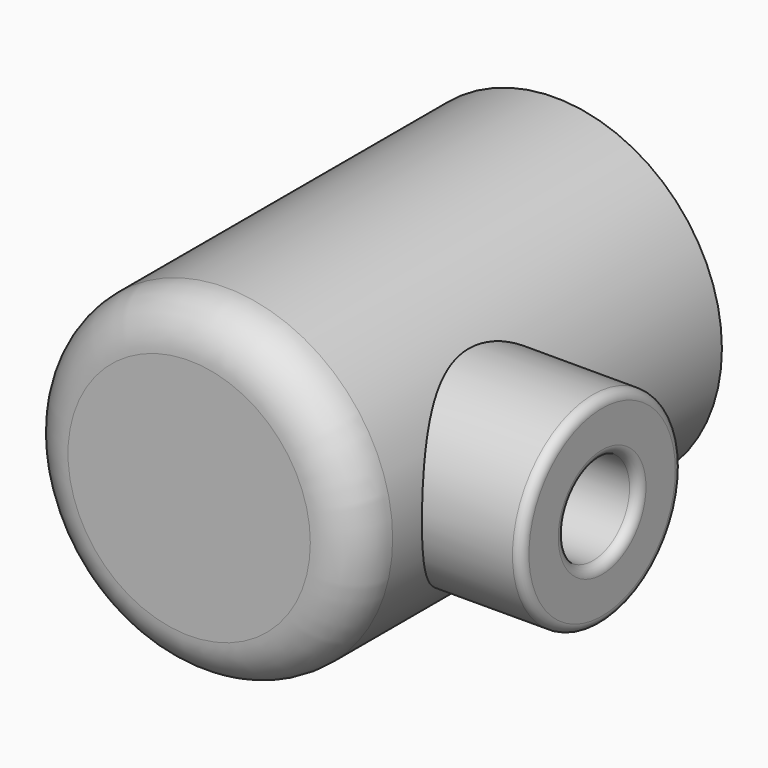
from build123d import *

# Parameters (mm, degrees)
F0_R           = 18.25
F0_R_2         = 15.25
F1_DEPTH       = 50
F2_R           = 18.25
F3_DEPTH       = 2
F4_R           = 5
F5_R           = 16.25
F6_DEPTH       = 10.5
F7_R           = 5
F8_DEPTH       = 18.251
F10_R          = 11
F10_R_2        = 5
F11_REACH      = 78.5136984722
F12_R          = 1
F14_DEPTH      = 8
F15_R          = 1.1
F16_ANGLE_BACK = 150
F16_ANGLE      = 300


with BuildPart() as f1:
    # F0 (on Front) → F1 (new body)
    with BuildSketch(Plane.XZ):
        Circle(F0_R)
        Circle(F0_R_2, mode=Mode.SUBTRACT)
    extrude(amount=F1_DEPTH)

    # F2 (on face) → F3 (join)
    with BuildSketch(Plane.XZ.offset(50)):
        Circle(F2_R)
    extrude(amount=-F3_DEPTH)

    # F4
    f4_edges = [f1.edges().sort_by_distance(p)[0] for p in [
        (-18.25, -50, 0),
    ]]
    fillet(f4_edges, radius=F4_R)

    # F5 (on face) → F6 (cut)
    with BuildSketch(Plane(origin=(0, 0, 0), x_dir=(-1, 0, 0), z_dir=(0, 1, 0))):
        Circle(F5_R)
    extrude(amount=-F6_DEPTH, mode=Mode.SUBTRACT)

    # F7 (on Right) → F8 (cut, through all)
    with BuildSketch(Plane.YZ):
        with Locations((-30, 0)):
            Circle(F7_R)
    extrude(amount=F8_DEPTH, mode=Mode.SUBTRACT)


with BuildPart() as f11:
    f11_end = f1.part.faces().sort_by_distance((-18.25, -22.5, 0))[0]
    # F10 (on offset) → F11 (new body, up to a face of F1 that its end follows)
    with BuildSketch(Plane.YZ.offset(29.15)):
        with Locations((-30, 0)):
            Circle(F10_R)
        with Locations((-30, 0)):
            Circle(F10_R_2, mode=Mode.SUBTRACT)
    f11_long = extrude(amount=-F11_REACH, mode=Mode.PRIVATE)
    add(split(f11_long, bisect_by=f11_end, keep=Keep.ALL, mode=Mode.PRIVATE).solids().sort_by_distance((29.15, -40.6888730163, 0))[0])

    # F12
    f12_edges = [f11.edges().sort_by_distance(p)[0] for p in [
        (29.15, -35, 0),
        (29.15, -41, 0),
    ]]
    fillet(f12_edges, radius=F12_R)


with BuildPart() as f1_1:
    add(f1.part)

    # F13 (on face) → F14 (join)
    with BuildSketch(Plane(origin=(0, -10.5, 0), x_dir=(-1, 0, 0), z_dir=(0, 1, 0))):
        with BuildLine():
            Line((13.6679369328, -1.5), (16.1806211253, -1.5))
            ThreePointArc((16.1806211253, -1.5), (16.25, 0), (16.1806211253, 1.5))
            Line((16.1806211253, 1.5), (13.6679369328, 1.5))
            ThreePointArc((13.6679369328, 1.5), (13.75, 0), (13.6679369328, -1.5))
        make_face()
    extrude(amount=F14_DEPTH)

    # F15 (on Top) → F16 (revolve)
    with BuildSketch(Plane.XY, mode=Mode.PRIVATE) as f16_sk:
        with Locations((16.25, -5.6)):
            Circle(F15_R)
    revolve(f16_sk.sketch.rotate(Axis((0, -13.1502728909, 0), (0, -1, 0)), -F16_ANGLE_BACK), axis=Axis((0, -13.1502728909, 0), (0, -1, 0)), revolution_arc=F16_ANGLE)


solid = Compound([f11.part, f1_1.part])
